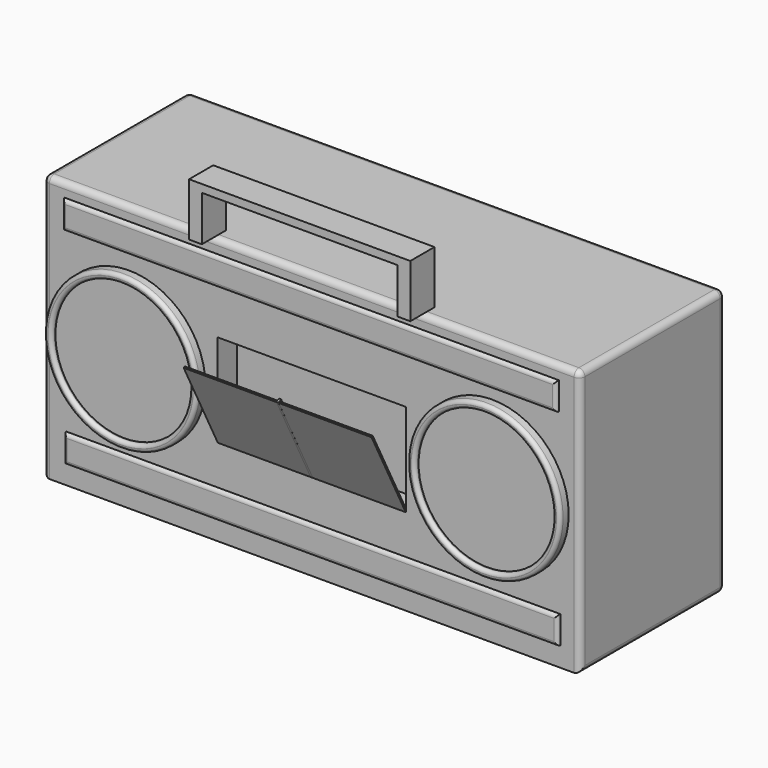
from build123d import *

# Parameters (mm, degrees)
F1_W          = 451.2749314308
F1_H          = 223.8389104605
F2_DEPTH      = 152.4
F0_W          = 158.242
F0_H          = 77.978
F3_DEPTH      = 20.32
F4_R          = 64.3254088221
F4_R_2        = 58.039602145
F4_R_3        = 58.0395969
F5_DEPTH      = 8.89
F6_DEPTH      = 4.826
F7_W          = 415.5984818935
F7_H          = 23.315563798
F8_DEPTH      = 2.794
F10_DEPTH     = 0.889
F12_DEPTH     = 78.994
F14_DEPTH     = 12.7
F15_R         = 3.0660512242
F16_T1_DEPTH  = 430.8682708909
F16_T3_DEPTH  = 38.5853527953
F16_T5_DEPTH  = 430.8682708909
F16_T7_DEPTH  = 38.5853527953
F17_T1_DEPTH  = 231.4589104605
F17_T3_DEPTH  = 213.6789104605
F17_T5_DEPTH  = 160.02
F17_T7_DEPTH  = 142.24
F17_T9_DEPTH  = 441.1149314308
F17_S13_W     = 5.1816
F17_S13_H     = 5.1816
F17_T14_DEPTH = 5.1816
F17_S19_W     = 5.1816
F17_S19_H     = 5.1816
F17_T20_DEPTH = 5.1816
F17_S25_W     = 5.1816
F17_S25_H     = 5.1816
F17_T26_DEPTH = 5.1816
F17_S31_W     = 5.1816
F17_S31_H     = 5.1816
F17_T32_DEPTH = 5.1816
F17_S37_W     = 5.1816
F17_S37_H     = 5.1816
F17_T38_DEPTH = 5.1816
F17_S43_W     = 5.1816
F17_S43_H     = 5.1816
F17_T44_DEPTH = 5.1816


# Not quite as in the source:
# - a fillet or chamfer that OpenCascade refuses, or shapes differently, is made with other operations: its cross-section is extruded or revolved along the edge and cut away or added


with BuildPart() as f2:
    # F1 (on Front) → F2 (new body)
    with BuildSketch(Plane.XZ):
        Rectangle(F1_W, F1_H)
    extrude(amount=-F2_DEPTH)

    # F0 (on Front) → F3 (cut)
    with BuildSketch(Plane.XZ):
        Rectangle(F0_W, F0_H)
    extrude(amount=-F3_DEPTH, mode=Mode.SUBTRACT)

    # F4 (on Front) → F5 (join)
    with BuildSketch(Plane.XZ):
        with Locations((-153.7030488253, 0)):
            Circle(F4_R)
        with Locations((-153.7030488253, 0)):
            Circle(F4_R_2, mode=Mode.SUBTRACT)
        with Locations((151.7204791307, 3.7095970474)):
            Circle(F4_R)
        with Locations((151.7204791307, 3.7095970474)):
            Circle(F4_R_3, mode=Mode.SUBTRACT)
    extrude(amount=F5_DEPTH)

    # F4 (on Front) → F6 (join)
    with BuildSketch(Plane.XZ):
        with Locations((151.7204791307, 3.7095970474)):
            Circle(F4_R_3)
        with Locations((-153.7030488253, 0)):
            Circle(F4_R_2)
    extrude(amount=F6_DEPTH)

    # F7 (on Front) → F8 (join)
    with BuildSketch(Plane.XZ):
        with Locations((0, 88.8867750764)):
            Rectangle(F7_W, F7_H)
        with Locations((1.256197691, -83.8089436293)):
            Rectangle(F7_W, F7_H)
    extrude(amount=F8_DEPTH)

    # F15
    f15_edges = [f2.edges().sort_by_distance(p)[0] for p in [
        (-211.742651, -8.89, 0),
        (-218.028458, -8.89, 0),
        (87.39507, -8.89, 3.709597),
        (93.680882, -8.89, 3.709597),
    ]]
    fillet(f15_edges, radius=F15_R)

    # F16: fillet of radius 3.0660512242 on 8 edges, made by hand

    # F16_s2 → F16_t1 (cut)
    with BuildSketch(Plane.YZ.offset(-215.4341354454)):
        with BuildLine():
            ThreePointArc((0, 100.5445569754), (-1.9901151157, 99.5602062788), (-2.794, 97.4905991759))
            Line((-2.794, 97.4905991759), (-2.794, 100.5445569754))
            Line((-2.794, 100.5445569754), (0, 100.5445569754))
        make_face()
        with BuildLine():
            ThreePointArc((0, 77.2289931774), (-1.9901151157, 78.213343874), (-2.794, 80.2829509769))
            Line((-2.794, 80.2829509769), (-2.794, 77.2289931774))
            Line((-2.794, 77.2289931774), (0, 77.2289931774))
        make_face()
    extrude(amount=F16_T1_DEPTH, mode=Mode.SUBTRACT)

    # F16_s4 → F16_t3 (cut)
    with BuildSketch(Plane.XY.offset(69.5940986788)):
        with BuildLine():
            ThreePointArc((-207.7992409468, 0), (-206.8148902502, -1.9901151157), (-204.7452831473, -2.794))
            Line((-204.7452831473, -2.794), (-207.7992409468, -2.794))
            Line((-207.7992409468, -2.794), (-207.7992409468, 0))
        make_face()
        with BuildLine():
            ThreePointArc((207.7992409468, 0), (206.8148902502, -1.9901151157), (204.7452831473, -2.794))
            Line((204.7452831473, -2.794), (207.7992409468, -2.794))
            Line((207.7992409468, -2.794), (207.7992409468, 0))
        make_face()
    extrude(amount=F16_T3_DEPTH, mode=Mode.SUBTRACT)

    # F16_s6 → F16_t5 (cut)
    with BuildSketch(Plane.YZ.offset(-214.1779377545)):
        with BuildLine():
            ThreePointArc((0, -72.1511617303), (-1.9901151157, -73.1355124269), (-2.794, -75.2051195298))
            Line((-2.794, -75.2051195298), (-2.794, -72.1511617303))
            Line((-2.794, -72.1511617303), (0, -72.1511617303))
        make_face()
        with BuildLine():
            ThreePointArc((0, -95.4667255282), (-1.9901151157, -94.4823748316), (-2.794, -92.4127677288))
            Line((-2.794, -92.4127677288), (-2.794, -95.4667255282))
            Line((-2.794, -95.4667255282), (0, -95.4667255282))
        make_face()
    extrude(amount=F16_T5_DEPTH, mode=Mode.SUBTRACT)

    # F16_s8 → F16_t7 (cut)
    with BuildSketch(Plane.XY.offset(-103.1016200269)):
        with BuildLine():
            ThreePointArc((209.0554386377, 0), (208.0710879411, -1.9901151157), (206.0014808383, -2.794))
            Line((206.0014808383, -2.794), (209.0554386377, -2.794))
            Line((209.0554386377, -2.794), (209.0554386377, 0))
        make_face()
        with BuildLine():
            ThreePointArc((-206.5430432558, 0), (-205.5586925592, -1.9901151157), (-203.4890854563, -2.794))
            Line((-203.4890854563, -2.794), (-206.5430432558, -2.794))
            Line((-206.5430432558, -2.794), (-206.5430432558, 0))
        make_face()
    extrude(amount=F16_T7_DEPTH, mode=Mode.SUBTRACT)

    # F17: fillet of radius 5.08 on 11 edges, made by hand

    # F17_s2 → F17_t1 (cut)
    with BuildSketch(Plane.XY.offset(-124.6194552302)):
        with BuildLine():
            ThreePointArc((-220.5574657154, 0), (-224.1495681638, 1.4878975516), (-225.6374657154, 5.08))
            Line((-225.6374657154, 5.08), (-225.6374657154, 0))
            Line((-225.6374657154, 0), (-220.5574657154, 0))
        make_face()
        with BuildLine():
            ThreePointArc((220.5574657154, 0), (224.1495681638, 1.4878975516), (225.6374657154, 5.08))
            Line((225.6374657154, 5.08), (225.6374657154, 0))
            Line((225.6374657154, 0), (220.5574657154, 0))
        make_face()
    extrude(amount=F17_T1_DEPTH, mode=Mode.SUBTRACT)

    # F17_s4 → F17_t3 (cut)
    with BuildSketch(Plane.XY.offset(-106.8394552302)):
        with BuildLine():
            ThreePointArc((-225.6374657154, 147.32), (-224.1495681638, 150.9121024484), (-220.5574657154, 152.4))
            Line((-220.5574657154, 152.4), (-225.6374657154, 152.4))
            Line((-225.6374657154, 152.4), (-225.6374657154, 147.32))
        make_face()
        with BuildLine():
            ThreePointArc((225.6374657154, 147.32), (224.1495681638, 150.9121024484), (220.5574657154, 152.4))
            Line((220.5574657154, 152.4), (225.6374657154, 152.4))
            Line((225.6374657154, 152.4), (225.6374657154, 147.32))
        make_face()
    extrude(amount=F17_T3_DEPTH, mode=Mode.SUBTRACT)

    # F17_s6 → F17_t5 (cut)
    with BuildSketch(Plane.XZ.offset(-147.32)):
        with BuildLine():
            ThreePointArc((225.6374657154, -106.8394552302), (224.1495681638, -110.4315576787), (220.5574657154, -111.9194552302))
            Line((220.5574657154, -111.9194552302), (225.6374657154, -111.9194552302))
            Line((225.6374657154, -111.9194552302), (225.6374657154, -106.8394552302))
        make_face()
        with BuildLine():
            ThreePointArc((-220.5574657154, -111.9194552302), (-224.1495681638, -110.4315576787), (-225.6374657154, -106.8394552302))
            Line((-225.6374657154, -106.8394552302), (-225.6374657154, -111.9194552302))
            Line((-225.6374657154, -111.9194552302), (-220.5574657154, -111.9194552302))
        make_face()
    extrude(amount=F17_T5_DEPTH, mode=Mode.SUBTRACT)

    # F17_s8 → F17_t7 (cut)
    with BuildSketch(Plane.XZ.offset(-147.32)):
        with BuildLine():
            ThreePointArc((225.6374657154, 106.8394552302), (224.1495681638, 110.4315576787), (220.5574657154, 111.9194552302))
            Line((220.5574657154, 111.9194552302), (225.6374657154, 111.9194552302))
            Line((225.6374657154, 111.9194552302), (225.6374657154, 106.8394552302))
        make_face()
        with BuildLine():
            ThreePointArc((-220.5574657154, 111.9194552302), (-224.1495681638, 110.4315576787), (-225.6374657154, 106.8394552302))
            Line((-225.6374657154, 106.8394552302), (-225.6374657154, 111.9194552302))
            Line((-225.6374657154, 111.9194552302), (-220.5574657154, 111.9194552302))
        make_face()
    extrude(amount=F17_T7_DEPTH, mode=Mode.SUBTRACT)

    # F17_s10 → F17_t9 (cut)
    with BuildSketch(Plane.YZ.offset(-220.5574657154)):
        with BuildLine():
            ThreePointArc((0, 106.8394552302), (1.4878975516, 110.4315576787), (5.08, 111.9194552302))
            Line((5.08, 111.9194552302), (0, 111.9194552302))
            Line((0, 111.9194552302), (0, 106.8394552302))
        make_face()
        with BuildLine():
            ThreePointArc((147.32, 111.9194552302), (150.9121024484, 110.4315576787), (152.4, 106.8394552302))
            Line((152.4, 106.8394552302), (152.4, 111.9194552302))
            Line((152.4, 111.9194552302), (147.32, 111.9194552302))
        make_face()
        with BuildLine():
            ThreePointArc((147.32, -111.9194552302), (150.9121024484, -110.4315576787), (152.4, -106.8394552302))
            Line((152.4, -106.8394552302), (152.4, -111.9194552302))
            Line((152.4, -111.9194552302), (147.32, -111.9194552302))
        make_face()
    extrude(amount=F17_T9_DEPTH, mode=Mode.SUBTRACT)


with BuildPart() as f10:
    # F9 (on Right) → F10 (new body, symmetric)
    with BuildSketch(Plane.YZ):
        Polygon((-36.0545791317, 31.2565839037), (0, -39.0403605998), (2.7178491377, -37.6464037572), (-33.3424917044, 32.6475856244), align=None)
    extrude(amount=F10_DEPTH, both=True)


with BuildPart() as f12:
    # F11 (on Right) → F12 (new body, symmetric)
    with BuildSketch(Plane.YZ):
        Polygon((-35.8992308868, 31.0243072869), (0, -39.041394805), (1.226429409, -38.4651481785), (-34.6939585845, 31.64184693), align=None)
    extrude(amount=F12_DEPTH, both=True)


with BuildPart() as f14:
    # F13 (on Front) → F14 (new body, symmetric)
    with BuildSketch(Plane.XZ):
        Polygon((-93.0209234357, 112.0174899697), (-82.2720825672, 112.0174899697), (-82.2720825672, 150.1174899697), (0, 150.1174899697), (82.2720825672, 150.1174899697), (82.2720825672, 112.0174899697), (93.0209234357, 112.0174899697), (93.0209234357, 150.1174899697), (93.0209234357, 156.6684097052), (0, 156.6684097052), (-93.0209234357, 156.6684097052), (-93.0209234357, 150.1174899697), align=None)
    extrude(amount=F14_DEPTH, both=True)


with BuildPart() as f17_tool12:
    # F17_s13 → F17_t14 (new body)
    with BuildSketch(Plane.XZ.offset(-5.08)):
        with Locations((-223.1482657154, 109.4302552302)):
            Rectangle(F17_S13_W, F17_S13_H)
    extrude(amount=F17_T14_DEPTH)

    # F17_s15 → F17_t16 (revolve, cut)
    with BuildSketch(Plane(origin=(-220.5574657154, 5.08, 106.8394552302), x_dir=(0.7071067812, 0, -0.7071067812), z_dir=(-0.7071067812, 0, -0.7071067812))):
        with BuildLine():
            ThreePointArc((0, -5.08), (5.08, 0), (0, 5.08))
            Line((0, 5.08), (0, -5.08))
        make_face()
    revolve(axis=Axis((-220.5574657154, 5.08, 106.8394552302), (0, -1, 0)), mode=Mode.SUBTRACT)


with BuildPart() as f2_1:
    add(f2.part)

    # F17_t11: cut F17_tool12
    add(f17_tool12.part, mode=Mode.SUBTRACT)


with BuildPart() as f17_tool18:
    # F17_s19 → F17_t20 (new body)
    with BuildSketch(Plane.XY.offset(106.8394552302)):
        with Locations((-223.1482657154, 149.9108)):
            Rectangle(F17_S19_W, F17_S19_H)
    extrude(amount=F17_T20_DEPTH)

    # F17_s21 → F17_t22 (revolve, cut)
    with BuildSketch(Plane(origin=(-220.5574657154, 147.32, 106.8394552302), x_dir=(0.7071067812, -0.7071067812, 0), z_dir=(-0.7071067812, -0.7071067812, 0))):
        with BuildLine():
            ThreePointArc((0, -5.08), (5.08, 0), (0, 5.08))
            Line((0, 5.08), (0, -5.08))
        make_face()
    revolve(axis=Axis((-220.5574657154, 147.32, 106.8394552302), (0, 0, 1)), mode=Mode.SUBTRACT)


with BuildPart() as f2_2:
    add(f2_1.part)

    # F17_t17: cut F17_tool18
    add(f17_tool18.part, mode=Mode.SUBTRACT)


with BuildPart() as f17_tool24:
    # F17_s25 → F17_t26 (new body)
    with BuildSketch(Plane.XY.offset(-106.8394552302)):
        with Locations((-223.1482657154, 149.9108)):
            Rectangle(F17_S25_W, F17_S25_H)
    extrude(amount=-F17_T26_DEPTH)

    # F17_s27 → F17_t28 (revolve, cut)
    with BuildSketch(Plane(origin=(-220.5574657154, 147.32, -106.8394552302), x_dir=(0.7071067812, -0.7071067812, 0), z_dir=(0.7071067812, 0.7071067812, 0))):
        with BuildLine():
            ThreePointArc((0, -5.08), (5.08, 0), (0, 5.08))
            Line((0, 5.08), (0, -5.08))
        make_face()
    revolve(axis=Axis((-220.5574657154, 147.32, -106.8394552302), (0, 0, -1)), mode=Mode.SUBTRACT)


with BuildPart() as f2_3:
    add(f2_2.part)

    # F17_t23: cut F17_tool24
    add(f17_tool24.part, mode=Mode.SUBTRACT)


with BuildPart() as f17_tool30:
    # F17_s31 → F17_t32 (new body)
    with BuildSketch(Plane.XZ.offset(-5.08)):
        with Locations((223.1482657154, 109.4302552302)):
            Rectangle(F17_S31_W, F17_S31_H)
    extrude(amount=F17_T32_DEPTH)

    # F17_s33 → F17_t34 (revolve, cut)
    with BuildSketch(Plane(origin=(220.5574657154, 5.08, 106.8394552302), x_dir=(-0.7071067812, 0, -0.7071067812), z_dir=(-0.7071067812, 0, 0.7071067812))):
        with BuildLine():
            ThreePointArc((0, -5.08), (5.08, 0), (0, 5.08))
            Line((0, 5.08), (0, -5.08))
        make_face()
    revolve(axis=Axis((220.5574657154, 5.08, 106.8394552302), (0, -1, 0)), mode=Mode.SUBTRACT)


with BuildPart() as f2_4:
    add(f2_3.part)

    # F17_t29: cut F17_tool30
    add(f17_tool30.part, mode=Mode.SUBTRACT)


with BuildPart() as f17_tool36:
    # F17_s37 → F17_t38 (new body)
    with BuildSketch(Plane.YZ.offset(220.5574657154)):
        with Locations((149.9108, -109.4302552302)):
            Rectangle(F17_S37_W, F17_S37_H)
    extrude(amount=F17_T38_DEPTH)

    # F17_s39 → F17_t40 (revolve, cut)
    with BuildSketch(Plane(origin=(220.5574657154, 147.32, -106.8394552302), x_dir=(0, -0.7071067812, 0.7071067812), z_dir=(0, 0.7071067812, 0.7071067812))):
        with BuildLine():
            ThreePointArc((0, -5.08), (5.08, 0), (0, 5.08))
            Line((0, 5.08), (0, -5.08))
        make_face()
    revolve(axis=Axis((220.5574657154, 147.32, -106.8394552302), (1, 0, 0)), mode=Mode.SUBTRACT)


with BuildPart() as f2_5:
    add(f2_4.part)

    # F17_t35: cut F17_tool36
    add(f17_tool36.part, mode=Mode.SUBTRACT)


with BuildPart() as f17_tool42:
    # F17_s43 → F17_t44 (new body)
    with BuildSketch(Plane.YZ.offset(220.5574657154)):
        with Locations((149.9108, 109.4302552302)):
            Rectangle(F17_S43_W, F17_S43_H)
    extrude(amount=F17_T44_DEPTH)

    # F17_s45 → F17_t46 (revolve, cut)
    with BuildSketch(Plane(origin=(220.5574657154, 147.32, 106.8394552302), x_dir=(0, -0.7071067812, -0.7071067812), z_dir=(0, -0.7071067812, 0.7071067812))):
        with BuildLine():
            ThreePointArc((0, -5.08), (5.08, 0), (0, 5.08))
            Line((0, 5.08), (0, -5.08))
        make_face()
    revolve(axis=Axis((220.5574657154, 147.32, 106.8394552302), (1, 0, 0)), mode=Mode.SUBTRACT)


with BuildPart() as f2_6:
    add(f2_5.part)

    # F17_t41: cut F17_tool42
    add(f17_tool42.part, mode=Mode.SUBTRACT)


solid = Compound([f10.part, f12.part, f14.part, f2_6.part])
